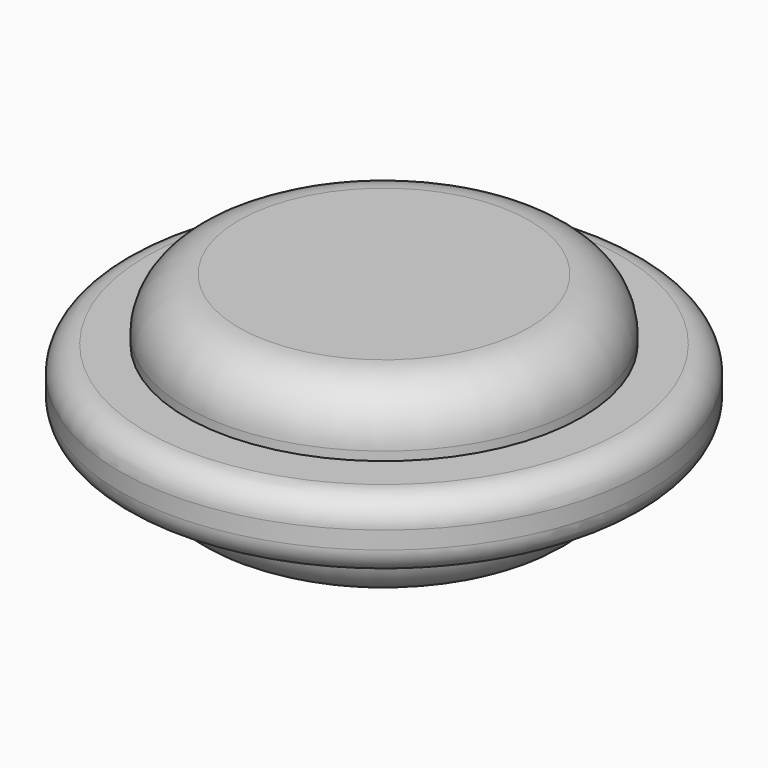
from build123d import *

# Parameters (mm, degrees)
F2_R     = 15
F2_R_2   = 11
F3_DEPTH = 2
F4_R     = 11.25
F5_DEPTH = 5.5
F6_R     = 3
F9_R     = 1.5


with BuildPart() as f3:
    # F2 (on Top) → F3 (new body, symmetric)
    with BuildSketch(Plane.XY):
        Circle(F2_R)
        Circle(F2_R_2, mode=Mode.SUBTRACT)
    extrude(amount=F3_DEPTH, both=True)


with BuildPart() as f5:
    # F4 (on Top) → F5 (new body, symmetric)
    with BuildSketch(Plane.XY):
        Circle(F4_R)
    extrude(amount=F5_DEPTH, both=True)

    # F6
    f6_edges = [f5.edges().sort_by_distance(p)[0] for p in [
        (-11.25, 0, 5.5),
        (-11.25, 0, -5.5),
    ]]
    fillet(f6_edges, radius=F6_R)


with BuildPart() as f7_1:
    # F7: copy of F3
    add(f3.part)


with BuildPart() as f5_1:
    add(f5.part)

    # F8: cut F7_1
    add(f7_1.part, mode=Mode.SUBTRACT)


with BuildPart() as f3_1:
    add(f3.part)

    # F9
    f9_edges = [f3_1.edges().sort_by_distance(p)[0] for p in [
        (-15, 0, -2),
        (15, 0, 0),
        (-15, 0, 2),
    ]]
    fillet(f9_edges, radius=F9_R)


solid = Compound([f5_1.part, f3_1.part])
